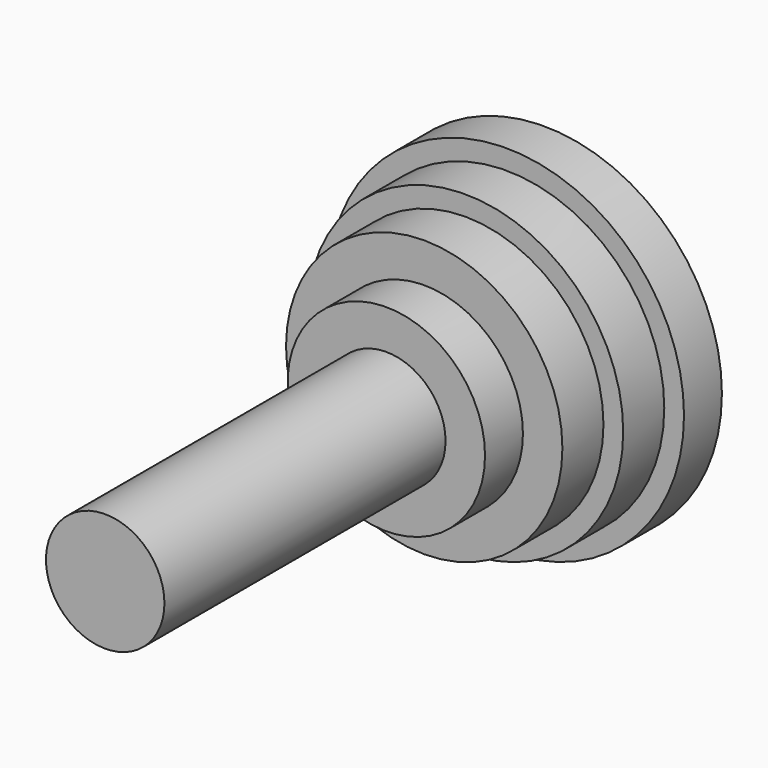
from build123d import *

# Parameters (mm, degrees)
F0_R     = 3.81
F1_DEPTH = 35.306
F2_R     = 6.35
F3_DEPTH = 12.7
F4_R     = 8.89
F5_DEPTH = 9.652
F6_R     = 10.16
F7_DEPTH = 6.35
F8_R     = 11.43
F9_DEPTH = 3.048


# Not quite as in the source:
# - the program builds the solid bodies; features that only make, move or delete a surface that nothing else refers to are left out


with BuildPart() as f1:
    # F0 (on Front) → F1 (new body)
    with BuildSketch(Plane.XZ):
        Circle(F0_R)
    extrude(amount=F1_DEPTH)

    # F2 (on Front) → F3 (join)
    with BuildSketch(Plane.XZ):
        Circle(F2_R)
    extrude(amount=F3_DEPTH)

    # F4 (on Front) → F5 (join)
    with BuildSketch(Plane.XZ):
        Circle(F4_R)
    extrude(amount=F5_DEPTH)

    # F6 (on Front) → F7 (join)
    with BuildSketch(Plane.XZ):
        Circle(F6_R)
    extrude(amount=F7_DEPTH)

    # F8 (on Front) → F9 (join)
    with BuildSketch(Plane.XZ):
        Circle(F8_R)
    extrude(amount=F9_DEPTH)


solid = f1.part
